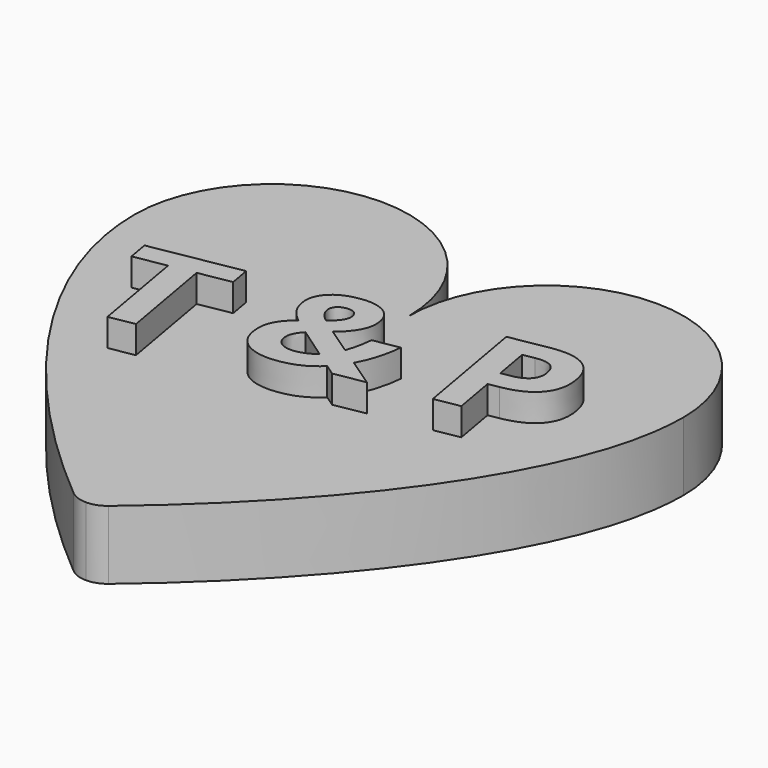
from build123d import *

# Parameters (mm, degrees)
F2_DEPTH     = 5
F1_TEXT_SIZE = 12.2291478975
F3_DEPTH     = 7


# Not quite as in the source:
# - Text() gives the source's letters only with a copy of the font that has no kerning and outlines rounded to 1/6400 em; it was checked with that copy


with BuildPart() as f2:
    # F0 (on Top) → F2 (new body)
    with BuildSketch(Plane.XY):
        with BuildLine():
            ThreePointArc((0, 0), (10, -10), (20, 0))
            ThreePointArc((20, 0), (10, 10), (0, 0))
        make_face()
        with BuildLine():
            add(Edge.make_bspline(
                [(1.2815378537, -28.9526889731), (10.8366087424, -20.9777990478), (20, -9.5725603981), (20, 0)],
                knots=[1.5411554017, 1.5411554017, 1.5411554017, 1.5411554017, 36.0555127546, 36.0555127546, 36.0555127546, 36.0555127546], degree=3))
            ThreePointArc((20, 0), (10, -10), (0, 0))
            Line((0, 0), (0, -22))
            Line((0, -22), (0, -29.41722138))
            ThreePointArc((0, -29.41722138), (0.6815661427, -29.2975052929), (1.2815378537, -28.9526889731))
        make_face()
        with BuildLine():
            ThreePointArc((-20, 0), (-10, -10), (0, 0))
            ThreePointArc((0, 0), (-10, 10), (-20, 0))
        make_face()
        with BuildLine():
            Line((0, -22), (0, 0))
            ThreePointArc((0, 0), (-10, -10), (-20, 0))
            add(Edge.make_bspline(
                [(-20, 0), (-20, -9.5725603981), (-10.8366087424, -20.9777990478), (-1.2815378537, -28.9526889731)],
                knots=[0, 0, 0, 0, 34.514357353, 34.514357353, 34.514357353, 34.514357353], degree=3))
            ThreePointArc((-1.2815378537, -28.9526889731), (-0.6815661427, -29.2975052929), (0, -29.41722138))
            Line((0, -29.41722138), (0, -22))
        make_face()
    extrude(amount=F2_DEPTH)

    # F1 (on Top) → F3 (join)
    with BuildSketch(Plane.XY):
        with Locations(Location((-13.5045301956, -14.263755149), (0, 0, 10))):
            Text('T & P', F1_TEXT_SIZE, font='Open Sans', font_style=FontStyle.BOLD, text_align=(TextAlign.LEFT, TextAlign.BOTTOM))
    extrude(amount=F3_DEPTH)


solid = f2.part
